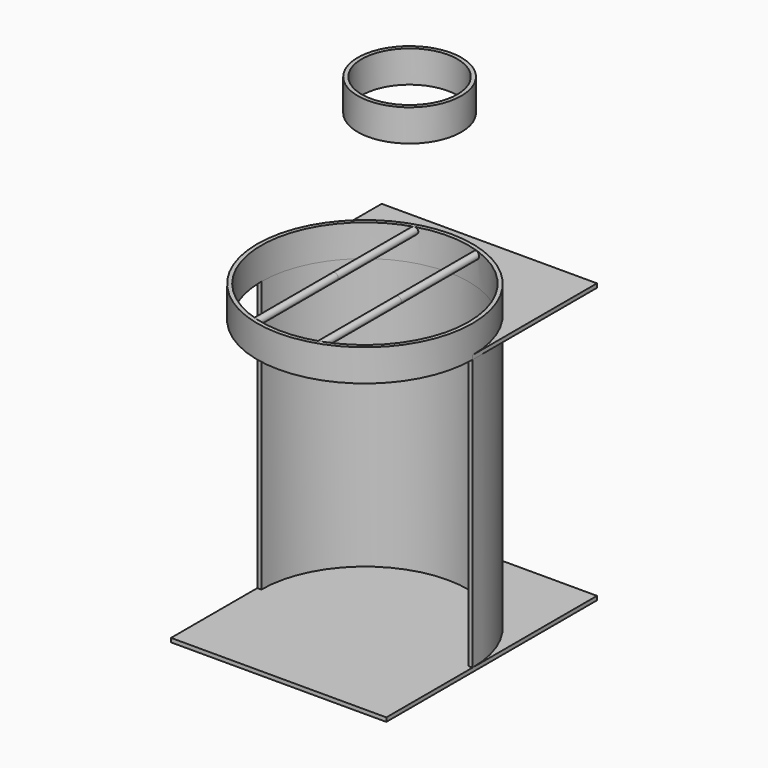
from build123d import *
from build123d import SkipClean  # not in build123d's __all__

# Parameters (mm, degrees)
F1_DEPTH       = 215.9
F2_W           = 171.45
F2_H           = 247.65
F3_DEPTH       = 3.175
F4_W           = 171.45
F4_H           = 37.9944009304
F5_DEPTH       = 25.4
F7_R           = 85.725
F7_R_2         = 82.55
F9_DEPTH       = 25.4
F10_R          = 41.275
F10_R_2        = 38.1
F11_DEPTH      = 25.4
F13_DEPTH      = 3.175
F14_R          = 2.8270786392
F14_R_2        = 2.8387354089
F15_DEPTH      = 79.7610810168
F15_DEPTH_BACK = 79.7610810168


# Not quite as in the source:
# - after a boolean that leaves OpenCascade's solid faulty, fix() repairs it


with BuildPart() as f1:
    # F0 (on Top) → F1 (new body)
    with BuildSketch(Plane.XY):
        with BuildLine():
            ThreePointArc((-82.55, 0), (0, 82.55), (82.55, 0))
            Line((82.55, 0), (85.725, 0))
            ThreePointArc((85.725, 0), (0, 85.725), (-85.725, 0))
            Line((-85.725, 0), (-82.55, 0))
        make_face()
    extrude(amount=F1_DEPTH)

    # F2 (on Top) → F3 (join)
    with BuildSketch(Plane.XY):
        Rectangle(F2_W, F2_H)
    extrude(amount=-F3_DEPTH)

    # F4 (on face) → F5 (cut)
    with BuildSketch(Plane.XY):
        with Locations((0, -104.8277995348)):
            Rectangle(F4_W, F4_H)
    extrude(amount=-F5_DEPTH, mode=Mode.SUBTRACT)

    # F7 (on offset) → F9 (join)
    with BuildSketch(Plane.XY.offset(215.9)):
        Circle(F7_R)
        Circle(F7_R_2, mode=Mode.SUBTRACT)
    with SkipClean():  # cleaning this boolean's faces spoils the solid; the shape is the same uncleaned
        extrude(amount=F9_DEPTH)

    # F12 (on offset) → F13 (join)
    with BuildSketch(Plane.XY.offset(215.9)):
        with BuildLine():
            Line((-85.725, 123.825), (-85.725, 0))
            ThreePointArc((-85.725, 0), (0, 85.725), (85.725, 0))
            Line((85.725, 0), (85.725, 123.825))
            Line((85.725, 123.825), (-85.725, 123.825))
        make_face()
    extrude(amount=F13_DEPTH)

    add(f1.part.fix(), mode=Mode.REPLACE)

    # F14 (on Front) → F15 (join, two sides)
    with BuildSketch(Plane.XZ) as f15_sk:
        with Locations((-24.103179574, 238.4221255779)):
            Circle(F14_R)
        with Locations((26.1746887118, 238.2481247187)):
            Circle(F14_R_2)
    extrude(amount=F15_DEPTH)
    extrude(f15_sk.sketch, amount=-F15_DEPTH_BACK)


with BuildPart() as f11:
    # F10 (on offset) → F11 (new body)
    with BuildSketch(Plane.XY.offset(368.3)):
        with Locations((0, 44.45)):
            Circle(F10_R)
        with Locations((0, 44.45)):
            Circle(F10_R_2, mode=Mode.SUBTRACT)
    extrude(amount=-F11_DEPTH)


solid = Compound([f1.part, f11.part])
